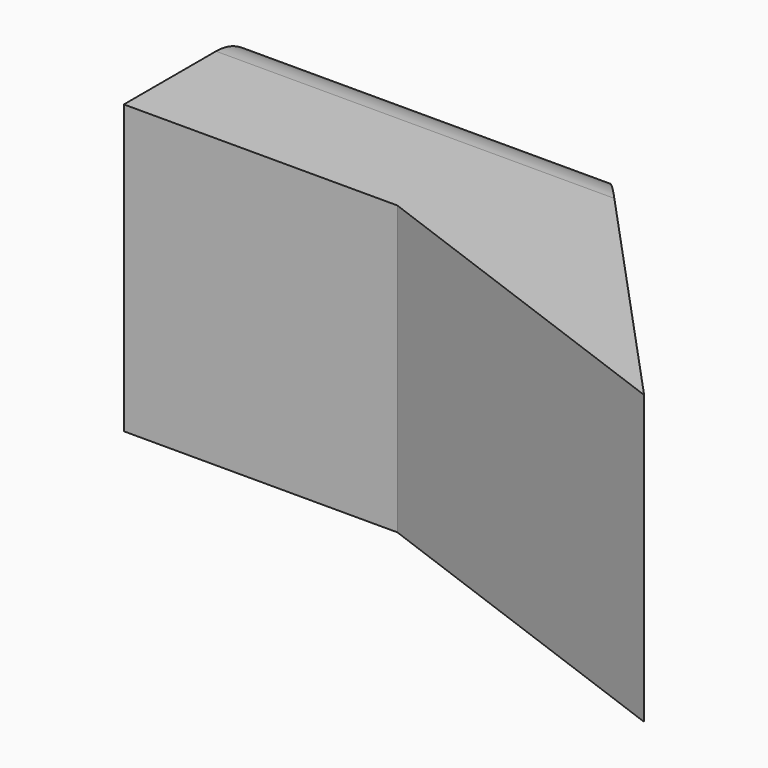
from build123d import *

# Parameters (mm, degrees)
F1_DEPTH = 25.4
F2_R     = 5.08
F3_R     = 5.08


# Not quite as in the source:
# - a feature names something its author has since deleted; it is built from what else it names


with BuildPart() as f1:
    # F0 (on Top) → F1 (new body)
    with BuildSketch(Plane.XY):
        Polygon((0, 15.24), (0, 0), (24.13, 0), (55.0936062386, -11.4706359327), (30.48, 15.24), align=None)
    extrude(amount=F1_DEPTH)

    # F2
    f2_edges = [f1.edges().sort_by_distance(p)[0] for p in [
        (15.24, 15.24, 25.4),
    ]]
    fillet(f2_edges, radius=F2_R)

    # F3
    f3_edges = [f1.edges().sort_by_distance(p)[0] for p in [
        (15.24, 15.24, 0),
    ]]
    fillet(f3_edges, radius=F3_R)


solid = f1.part
